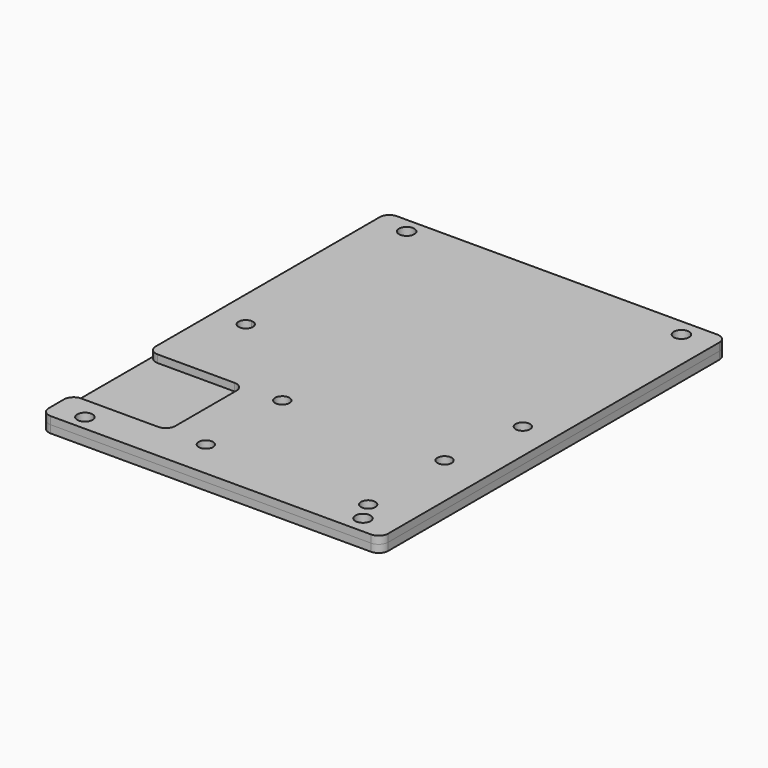
from build123d import *

# Parameters (mm, degrees)
F0_R     = 1.6
F1_DEPTH = 1.6
F2_R     = 2
F3_R     = 1.6
F3_R_2   = 1.5
F4_DEPTH = 1.6
F5_R     = 2


# Not quite as in the source:
# - a feature names something its author has since deleted; it is built from what else it names


with BuildPart() as f1:
    # F0 (on Top) → F1 (new body)
    with BuildSketch(Plane.XY):
        Polygon((22.86, -45.339), (35.56, -45.339), (35.56, 45.339), (22.86, 45.339), (-22.86, 45.339), (-35.56, 45.339), (-35.56, -45.339), (-22.86, -45.339), align=None)
        with Locations((-28.956, -42.126997942)):
            Circle(F0_R, mode=Mode.SUBTRACT)
        with Locations((28.956, -41.694)):
            Circle(F0_R, mode=Mode.SUBTRACT)
        with Locations((-28.956, 42.126997942)):
            Circle(F0_R, mode=Mode.SUBTRACT)
        with Locations((28.956, 41.694)):
            Circle(F0_R, mode=Mode.SUBTRACT)
    extrude(amount=-F1_DEPTH)

    # F2
    f2_edges = [f1.edges().sort_by_distance(p)[0] for p in [
        (-35.56, 45.339, -0.8),
        (35.56, 45.339, -0.8),
        (-35.56, -45.339, -0.8),
        (35.56, -45.339, -0.8),
    ]]
    fillet(f2_edges, radius=F2_R)


with BuildPart() as f4:
    # F3 (on face) → F4 (new body)
    with BuildSketch(Plane.XY):
        with BuildLine():
            Line((-35.56, -17.339), (-19.8256308937, -17.339))
            Line((-19.8256308937, -17.339), (-15.44, -17.339))
            Line((-15.44, -17.339), (-8.94, -17.339))
            ThreePointArc((-8.94, -17.339), (-7.44, -15.839), (-5.94, -17.339))
            Line((-5.94, -17.339), (25.06, -17.339))
            ThreePointArc((25.06, -17.339), (26.56, -15.839), (28.06, -17.339))
            Line((28.06, -17.339), (34.56, -17.339))
            Line((34.56, -17.339), (34.56, -37.339))
            Line((34.56, -37.339), (28.06, -37.339))
            ThreePointArc((28.06, -37.339), (26.56, -38.839), (25.06, -37.339))
            Line((25.06, -37.339), (-5.94, -37.339))
            ThreePointArc((-5.94, -37.339), (-7.44, -38.839), (-8.94, -37.339))
            Line((-8.94, -37.339), (-15.44, -37.339))
            Line((-15.44, -37.339), (-35.56, -37.339))
            Line((-35.56, -37.339), (-35.56, -45.339))
            Line((-35.56, -45.339), (-22.86, -45.339))
            Line((-22.86, -45.339), (22.86, -45.339))
            Line((22.86, -45.339), (35.56, -45.339))
            Line((35.56, -45.339), (35.56, 45.339))
            Line((35.56, 45.339), (22.86, 45.339))
            Line((22.86, 45.339), (-22.86, 45.339))
            Line((-22.86, 45.339), (-35.56, 45.339))
            Line((-35.56, 45.339), (-35.56, -17.339))
        make_face()
        with Locations((-28.956, -42.126997942)):
            Circle(F3_R, mode=Mode.SUBTRACT)
        with BuildLine():
            ThreePointArc((-27.456, 0), (-30.0166601718, -1.0606601718), (-28.956, 1.5))
            ThreePointArc((-28.956, 1.5), (-27.8953398282, 1.0606601718), (-27.456, 0))
        make_face(mode=Mode.SUBTRACT)
        with Locations((28.956, -41.694)):
            Circle(F3_R, mode=Mode.SUBTRACT)
        with Locations((29.0846601129, 0)):
            Circle(F3_R_2, mode=Mode.SUBTRACT)
        with BuildLine():
            ThreePointArc((-27.356, 42.126997942), (-27.8246291501, 40.9956270921), (-28.956, 40.526997942))
            ThreePointArc((-28.956, 40.526997942), (-30.0873708499, 43.2583687919), (-27.356, 42.126997942))
        make_face(mode=Mode.SUBTRACT)
        with BuildLine():
            ThreePointArc((27.4999902592, 17.0231461525), (27.4999975648, 17.0115730773), (27.5, 17))
            ThreePointArc((27.5, 17), (13.75, -6.8156986041), (-13.75, -6.8156986041))
            ThreePointArc((-13.75, -6.8156986041), (-23.8214830338, 3.2600237965), (-27.4999902592, 17.0231461525))
            ThreePointArc((-27.4999902592, 17.0231461525), (0, 44.5), (27.4999902592, 17.0231461525))
        make_face(mode=Mode.SUBTRACT)
        with Locations((28.956, 41.694)):
            Circle(F3_R, mode=Mode.SUBTRACT)
        with BuildLine():
            ThreePointArc((-13.75, -6.8156986041), (13.75, -6.8156986041), (27.5, 17))
            ThreePointArc((27.5, 17), (27.4999975648, 17.0115730773), (27.4999902592, 17.0231461525))
            Line((27.4999902592, 17.0231461525), (-27.4999902592, 17.0231461525))
            ThreePointArc((-27.4999902592, 17.0231461525), (-23.8214830338, 3.2600237965), (-13.75, -6.8156986041))
        make_face()
        with BuildLine():
            Line((-27.4999902592, 17.0231461525), (27.4999902592, 17.0231461525))
            ThreePointArc((27.4999902592, 17.0231461525), (0, 44.5), (-27.4999902592, 17.0231461525))
        make_face()
        with BuildLine():
            Line((-8.94, -17.339), (-15.44, -17.339))
            Line((-15.44, -17.339), (-15.44, -37.339))
            Line((-15.44, -37.339), (-8.94, -37.339))
            ThreePointArc((-8.94, -37.339), (-7.44, -35.839), (-5.94, -37.339))
            Line((-5.94, -37.339), (25.06, -37.339))
            ThreePointArc((25.06, -37.339), (26.56, -35.839), (28.06, -37.339))
            Line((28.06, -37.339), (34.56, -37.339))
            Line((34.56, -37.339), (34.56, -17.339))
            Line((34.56, -17.339), (28.06, -17.339))
            ThreePointArc((28.06, -17.339), (26.56, -18.839), (25.06, -17.339))
            Line((25.06, -17.339), (-5.94, -17.339))
            ThreePointArc((-5.94, -17.339), (-7.44, -18.839), (-8.94, -17.339))
        make_face()
    extrude(amount=F4_DEPTH)

    # F5
    f5_edges = [f4.edges().sort_by_distance(p)[0] for p in [
        (-15.44, -17.339, 0.8),
        (-35.56, -17.339, 0.8),
        (-35.56, -37.339, 0.8),
        (-15.44, -37.339, 0.8),
        (-35.56, -45.339, 0.8),
        (35.56, 45.339, 0.8),
        (-35.56, 45.339, 0.8),
        (35.56, -45.339, 0.8),
    ]]
    fillet(f5_edges, radius=F5_R)


solid = Compound([f1.part, f4.part])
